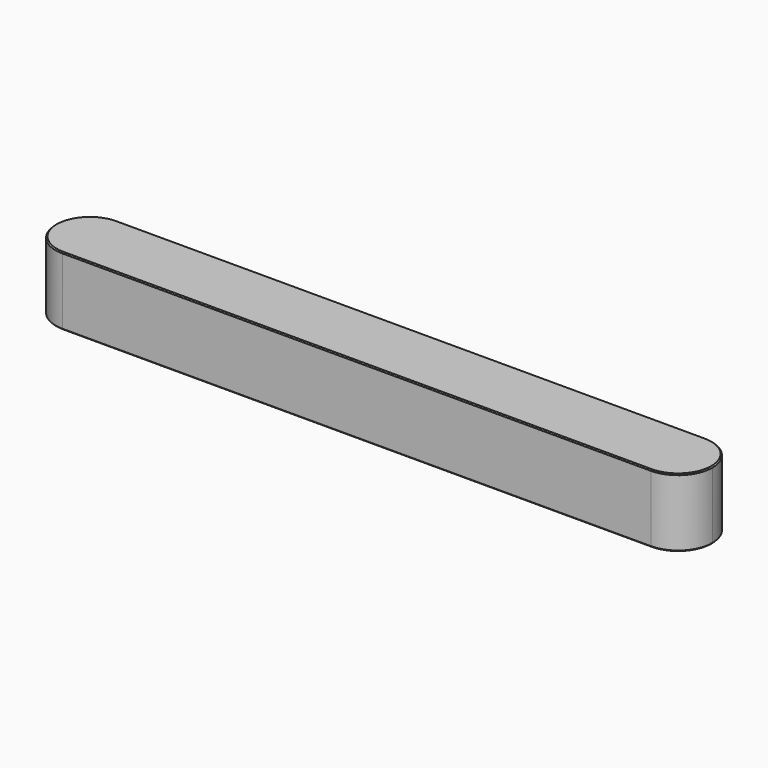
from build123d import *

# Parameters (mm, degrees)
F0_W     = 152.4
F0_H     = 15.875
F1_DEPTH = 15.875
F2_R     = 7.93749
F3_SIZE  = 0.254


# Not quite as in the source:
# - a fillet or chamfer is up to 0.001 mm smaller than in the source, because OpenCascade refuses the exact size


with BuildPart() as f1:
    # F0 (on Top) → F1 (new body)
    with BuildSketch(Plane.XY):
        Rectangle(F0_W, F0_H)
    extrude(amount=F1_DEPTH)

    # F2 (radius 7.9375 in the source; OpenCascade refuses exactly that, so slightly less here)
    f2_edges = [f1.edges().sort_by_distance(p)[0] for p in [
        (-76.2, 7.9375, 7.9375),
        (-76.2, -7.9375, 7.9375),
        (76.2, -7.9375, 7.9375),
        (76.2, 7.9375, 7.9375),
    ]]
    fillet(f2_edges, radius=F2_R)

    # F3
    f3_edges = [f1.edges().sort_by_distance(p)[0] for p in [
        (0, -7.9375, 0),
        (-73.875163, -5.612663, 0),
        (73.875163, -5.612663, 0),
        (-76.2, 0, 0),
        (76.2, 0, 0),
        (-73.875163, 5.612663, 0),
        (73.875163, 5.612663, 0),
        (0, 7.9375, 0),
        (0, -7.9375, 15.875),
        (-73.875163, -5.612663, 15.875),
        (73.875163, -5.612663, 15.875),
        (-76.2, 0, 15.875),
        (76.2, 0, 15.875),
        (-73.875163, 5.612663, 15.875),
        (73.875163, 5.612663, 15.875),
        (0, 7.9375, 15.875),
    ]]
    chamfer(f3_edges, length=F3_SIZE)


solid = f1.part
